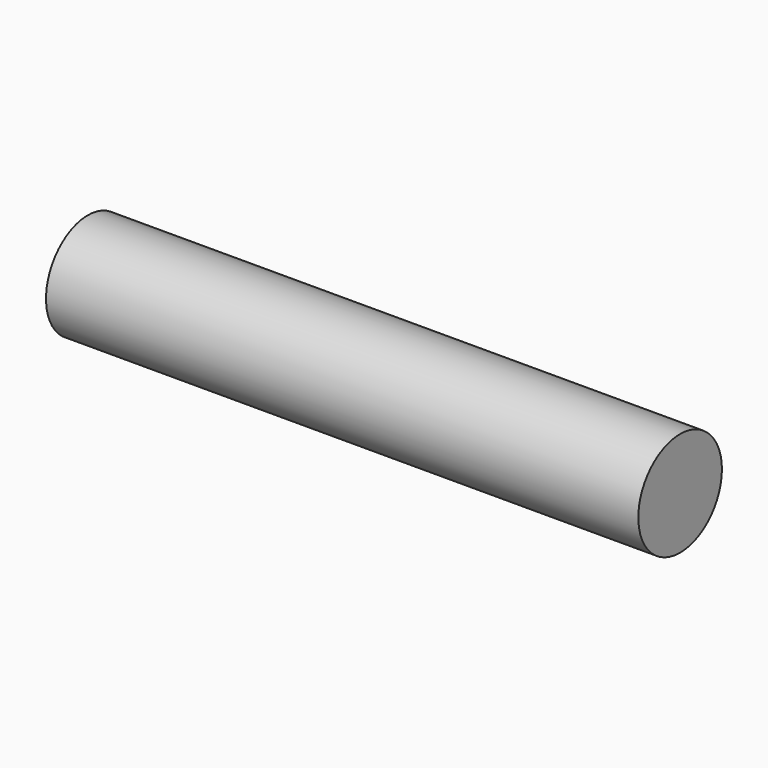
from build123d import *

# Parameters (mm, degrees)
F0_R     = 38.1
F2_DEPTH = 431.8


# Not quite as in the source:
# - the program builds the solid bodies; features that only make, move or delete a surface that nothing else refers to are left out


with BuildPart() as f2:
    # F0 (on Right) → F2 (new body)
    with BuildSketch(Plane.YZ):
        Circle(F0_R)
    extrude(amount=F2_DEPTH)


solid = f2.part
